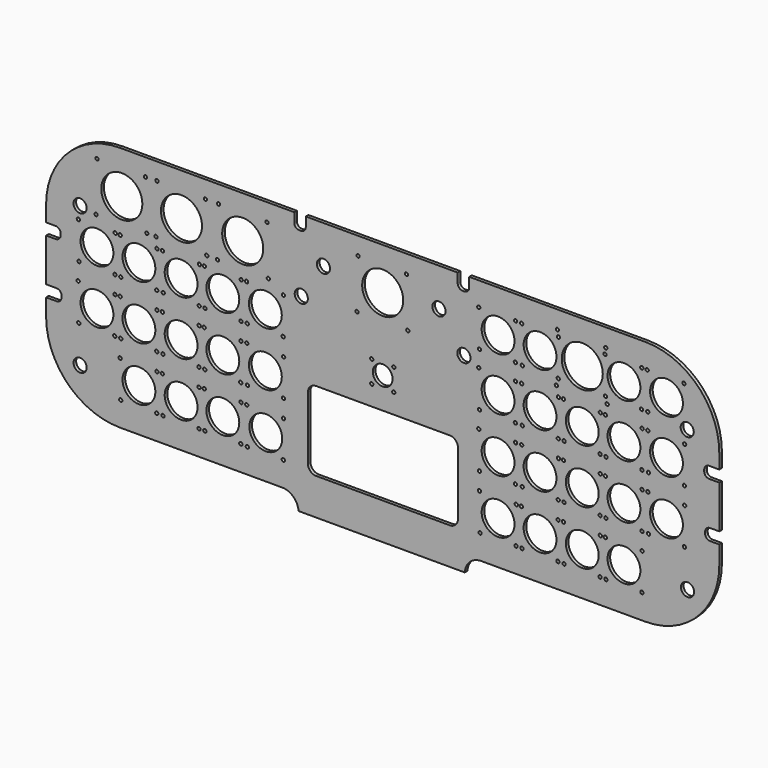
from build123d import *

# Parameters (mm, degrees)
F0_W           = 410
F0_H           = 150
F1_DEPTH       = 1
F1_DEPTH_BACK  = 1
F2_R           = 45
F3_R           = 45
F4_R           = 45
F5_W           = 101.2708619237
F5_H           = 20.8901241422
F6_DEPTH       = 1
F6_DEPTH_BACK  = 1
F7_T1_DEPTH    = 2
F8_T1_DEPTH    = 2
F13_R          = 4
F14_DEPTH      = 28.48665
F14_DEPTH_BACK = 25
F9_R           = 12.5
F9_R_2         = 6
F9_R_3         = 10
F9_W           = 91.4226509631
F9_H           = 48.2046687976
F15_DEPTH      = 25
F15_DEPTH_BACK = 25
F16_DEPTH      = 50
F16_DEPTH_BACK = 50
F19_D          = 2
F19_DEPTH      = 20
F19_TIP        = 0.600860619
F20_D          = 2
F20_DEPTH      = 20
F20_TIP        = 0.600860619
F21_D          = 2
F21_DEPTH      = 20
F21_TIP        = 0.600860619
F22_R          = 5


# Not quite as in the source:
# - a fillet or chamfer that OpenCascade refuses, or shapes differently, is made with other operations: its cross-section is extruded or revolved along the edge and cut away or added


with BuildPart() as f1:
    # F0 (on Front) → F1 (new body, two sides)
    with BuildSketch(Plane.XZ) as f1_sk:
        Rectangle(F0_W, F0_H)
    extrude(amount=F1_DEPTH)
    extrude(f1_sk.sketch, amount=-F1_DEPTH_BACK)

    # F2
    f2_edges = [f1.edges().sort_by_distance(p)[0] for p in [
        (-205, 0, 75),
        (-205, 0, -75),
    ]]
    fillet(f2_edges, radius=F2_R)

    # F3
    f3_edges = [f1.edges().sort_by_distance(p)[0] for p in [
        (205, 0, 75),
    ]]
    fillet(f3_edges, radius=F3_R)

    # F4
    f4_edges = [f1.edges().sort_by_distance(p)[0] for p in [
        (205, 0, -75),
    ]]
    fillet(f4_edges, radius=F4_R)

    # F5 (on Front) → F6 (join, two sides)
    with BuildSketch(Plane.XZ) as f6_sk:
        with Locations((-0.6414987147, -73.9290080965)):
            Rectangle(F5_W, F5_H)
    extrude(amount=F6_DEPTH)
    extrude(f6_sk.sketch, amount=-F6_DEPTH_BACK)

    # F7: fillet of radius 10 on 1 edges, made by hand

    # F7_s2 → F7_t1 (join)
    with BuildSketch(Plane.XZ.offset(-1)):
        with BuildLine():
            ThreePointArc((-61.2573210439, -75), (-54.4111286103, -77.7109912085), (-51.2769296765, -84.3740701675))
            Line((-51.2769296765, -84.3740701675), (-51.2769296765, -75))
            Line((-51.2769296765, -75), (-61.2573210439, -75))
        make_face()
    extrude(amount=F7_T1_DEPTH)

    # F8: fillet of radius 10 on 1 edges, made by hand

    # F8_s2 → F8_t1 (join)
    with BuildSketch(Plane.XZ.offset(-1)):
        with BuildLine():
            ThreePointArc((49.9939322472, -84.3740701675), (53.1281311809, -77.7109912085), (59.9743236145, -75))
            Line((59.9743236145, -75), (49.9939322472, -75))
            Line((49.9939322472, -75), (49.9939322472, -84.3740701675))
        make_face()
    extrude(amount=F8_T1_DEPTH)

    # F13 (on offset) → F14 (cut, two sides)
    with BuildSketch(Plane.XZ.offset(-1)) as f14_sk:
        with Locations((-184.3019276857, 36.01404652)):
            Circle(F13_R)
        with Locations((-184.2796504498, -49.4647398591)):
            Circle(F13_R)
        with Locations((-36.0691249371, 51.8314018846)):
            Circle(F13_R)
        with Locations((-49.5743155479, 31.3860401511)):
            Circle(F13_R)
        with Locations((34.2704169452, 51.8314018846)):
            Circle(F13_R)
        with Locations((49.4637563825, 31.7611843348)):
            Circle(F13_R)
        with Locations((185.4535341263, 36.2629145384)):
            Circle(F13_R)
        with Locations((185.6411099434, -49.4575425982)):
            Circle(F13_R)
    extrude(amount=F14_DEPTH, mode=Mode.SUBTRACT)
    extrude(f14_sk.sketch, amount=-F14_DEPTH_BACK, mode=Mode.SUBTRACT)

    # F9 (on Front) → F15 (cut, two sides)
    with BuildSketch(Plane.XZ) as f15_sk:
        with Locations((0, 49.3269376457)):
            Circle(F9_R)
        with Locations((0, 5.0263302401)):
            Circle(F9_R_2)
        with Locations((-158.883143139, 49.3269376457)):
            Circle(F9_R)
        with Locations((-122.5375886227, 49.3269376457)):
            Circle(F9_R)
        with Locations((-85.2427311078, 49.3269376457)):
            Circle(F9_R)
        with Locations((172.8430779376, 17.2050477801)):
            Circle(F9_R_3)
        with Locations((172.8430779376, -15.7630319912)):
            Circle(F9_R_3)
        with Locations((146.9427224634, -48.7311117624)):
            Circle(F9_R_3)
        with Locations((146.9427224634, 17.2050477801)):
            Circle(F9_R_3)
        with Locations((146.9427224634, -15.7630319912)):
            Circle(F9_R_3)
        with Locations((121.5410116401, -48.7311117624)):
            Circle(F9_R_3)
        with Locations((121.5410116401, 17.2050477801)):
            Circle(F9_R_3)
        with Locations((121.5410116401, -15.7630319912)):
            Circle(F9_R_3)
        with Locations((95.8335487816, -48.7311117624)):
            Circle(F9_R_3)
        with Locations((95.8335487816, 17.2050477801)):
            Circle(F9_R_3)
        with Locations((95.8335487816, -15.7630319912)):
            Circle(F9_R_3)
        with Locations((70.2727413384, -48.7311117624)):
            Circle(F9_R_3)
        with Locations((70.2727413384, 17.2050477801)):
            Circle(F9_R_3)
        with Locations((70.2727413384, -15.7630319912)):
            Circle(F9_R_3)
        with Locations((172.8430779376, 49.4541965136)):
            Circle(F9_R_3)
        with Locations((146.9427224634, 49.4541965136)):
            Circle(F9_R_3)
        with Locations((121.5410116401, 49.4541965136)):
            Circle(F9_R)
        with Locations((95.8335487816, 49.4541965136)):
            Circle(F9_R_3)
        with Locations((70.2727413384, 49.4541965136)):
            Circle(F9_R_3)
        with Locations((-71.4465556458, 17.2050477801)):
            Circle(F9_R_3)
        with Locations((-71.4465556458, -15.7630319912)):
            Circle(F9_R_3)
        with Locations((-97.3469263927, -48.7311117624)):
            Circle(F9_R_3)
        with Locations((-97.3469263927, 17.2050477801)):
            Circle(F9_R_3)
        with Locations((-97.3469263927, -15.7630319912)):
            Circle(F9_R_3)
        with Locations((-122.7486547945, -48.7311117624)):
            Circle(F9_R_3)
        with Locations((-122.7486547945, 17.2050477801)):
            Circle(F9_R_3)
        with Locations((-122.7486547945, -15.7630319912)):
            Circle(F9_R_3)
        with Locations((-148.4561388125, -48.7311117624)):
            Circle(F9_R_3)
        with Locations((-148.4561388125, 17.2050477801)):
            Circle(F9_R_3)
        with Locations((-148.4561388125, -15.7630319912)):
            Circle(F9_R_3)
        with Locations((-174.0169717099, 17.2050477801)):
            Circle(F9_R_3)
        with Locations((-174.0169717099, -15.7630319912)):
            Circle(F9_R_3)
        with Locations((-71.195551245, -48.846316319)):
            Circle(F9_R_3)
        with Locations((0.1603271812, -37.9611137323)):
            Rectangle(F9_W, F9_H)
    extrude(amount=F15_DEPTH, mode=Mode.SUBTRACT)
    extrude(f15_sk.sketch, amount=-F15_DEPTH_BACK, mode=Mode.SUBTRACT)

    # F11 (on offset) → F16 (cut, two sides)
    with BuildSketch(Plane.XZ.offset(1)) as f16_sk:
        with BuildLine():
            Line((-199.1314905395, 20.3550893723), (-210.3814848701, 20.3550893723))
            ThreePointArc((-210.3814848701, 20.3550893723), (-212.5028052137, 19.4764097158), (-213.3814848701, 17.3550893723))
            Line((-213.3814848701, 17.3550893723), (-213.3814848701, 16.3550893723))
            ThreePointArc((-213.3814848701, 16.3550893723), (-212.5028052137, 14.2337690287), (-210.3814848701, 13.3550893723))
            Line((-210.3814848701, 13.3550893723), (-199.1314905395, 13.3550893723))
            ThreePointArc((-199.1314905395, 13.3550893723), (-197.010170196, 14.2337690287), (-196.1314905395, 16.3550893723))
            Line((-196.1314905395, 16.3550893723), (-196.1314905395, 17.3550893723))
            ThreePointArc((-196.1314905395, 17.3550893723), (-197.010170196, 19.4764097158), (-199.1314905395, 20.3550893723))
        make_face()
        with BuildLine():
            Line((-198.5897086968, -12.8095770695), (-209.8397030274, -12.8095770695))
            ThreePointArc((-209.8397030274, -12.8095770695), (-211.961023371, -13.6882567259), (-212.8397030274, -15.8095770695))
            Line((-212.8397030274, -15.8095770695), (-212.8397030274, -16.8095770695))
            ThreePointArc((-212.8397030274, -16.8095770695), (-211.961023371, -18.930897413), (-209.8397030274, -19.8095770695))
            Line((-209.8397030274, -19.8095770695), (-198.5897086968, -19.8095770695))
            ThreePointArc((-198.5897086968, -19.8095770695), (-196.4683883532, -18.930897413), (-195.5897086968, -16.8095770695))
            Line((-195.5897086968, -16.8095770695), (-195.5897086968, -15.8095770695))
            ThreePointArc((-195.5897086968, -15.8095770695), (-196.4683883532, -13.6882567259), (-198.5897086968, -12.8095770695))
        make_face()
        with BuildLine():
            Line((210.0697169493, 21.1949502202), (198.8197226187, 21.1949502202))
            ThreePointArc((198.8197226187, 21.1949502202), (196.6984022751, 20.3162705637), (195.8197226187, 18.1949502202))
            Line((195.8197226187, 18.1949502202), (195.8197226187, 17.1949502202))
            ThreePointArc((195.8197226187, 17.1949502202), (196.6984022751, 15.0736298766), (198.8197226187, 14.1949502202))
            Line((198.8197226187, 14.1949502202), (210.0697169493, 14.1949502202))
            ThreePointArc((210.0697169493, 14.1949502202), (212.1910372928, 15.0736298766), (213.0697169493, 17.1949502202))
            Line((213.0697169493, 17.1949502202), (213.0697169493, 18.1949502202))
            ThreePointArc((213.0697169493, 18.1949502202), (212.1910372928, 20.3162705637), (210.0697169493, 21.1949502202))
        make_face()
        with BuildLine():
            Line((210.611498792, -11.9697162216), (199.3615044614, -11.9697162216))
            ThreePointArc((199.3615044614, -11.9697162216), (197.2401841178, -12.848395878), (196.3615044614, -14.9697162216))
            Line((196.3615044614, -14.9697162216), (196.3615044614, -15.9697162216))
            ThreePointArc((196.3615044614, -15.9697162216), (197.2401841178, -18.0910365651), (199.3615044614, -18.9697162216))
            Line((199.3615044614, -18.9697162216), (210.611498792, -18.9697162216))
            ThreePointArc((210.611498792, -18.9697162216), (212.7328191355, -18.0910365651), (213.611498792, -15.9697162216))
            Line((213.611498792, -15.9697162216), (213.611498792, -14.9697162216))
            ThreePointArc((213.611498792, -14.9697162216), (212.7328191355, -12.848395878), (210.611498792, -11.9697162216))
        make_face()
        with BuildLine():
            Line((-49.8431804255, 85.1224669314), (-50.8431804255, 85.1224669314))
            ThreePointArc((-50.8431804255, 85.1224669314), (-52.964500769, 84.2437872749), (-53.8431804255, 82.1224669314))
            Line((-53.8431804255, 82.1224669314), (-53.8431804255, 69.3415574527))
            ThreePointArc((-53.8431804255, 69.3415574527), (-52.964500769, 67.2202371091), (-50.8431804255, 66.3415574527))
            Line((-50.8431804255, 66.3415574527), (-49.8431804255, 66.3415574527))
            ThreePointArc((-49.8431804255, 66.3415574527), (-47.7218600819, 67.2202371091), (-46.8431804255, 69.3415574527))
            Line((-46.8431804255, 69.3415574527), (-46.8431804255, 82.1224669314))
            ThreePointArc((-46.8431804255, 82.1224669314), (-47.7218600819, 84.2437872749), (-49.8431804255, 85.1224669314))
        make_face()
        with BuildLine():
            Line((49.6914108768, 84.9684671557), (48.6914108768, 84.9684671557))
            ThreePointArc((48.6914108768, 84.9684671557), (46.5700905333, 84.0897874993), (45.6914108768, 81.9684671557))
            Line((45.6914108768, 81.9684671557), (45.6914108768, 69.187557677))
            ThreePointArc((45.6914108768, 69.187557677), (46.5700905333, 67.0662373335), (48.6914108768, 66.187557677))
            Line((48.6914108768, 66.187557677), (49.6914108768, 66.187557677))
            ThreePointArc((49.6914108768, 66.187557677), (51.8127312204, 67.0662373335), (52.6914108768, 69.187557677))
            Line((52.6914108768, 69.187557677), (52.6914108768, 81.9684671557))
            ThreePointArc((52.6914108768, 81.9684671557), (51.8127312204, 84.0897874993), (49.6914108768, 84.9684671557))
        make_face()
    extrude(amount=-F16_DEPTH, mode=Mode.SUBTRACT)
    extrude(f16_sk.sketch, amount=F16_DEPTH_BACK, mode=Mode.SUBTRACT)

    # F19
    with Locations(Plane(origin=(0, 1, 0), x_dir=(-1, 0, 0), z_dir=(0, 1, 0))):
        with Locations((173.9457249641, 64.6309927106), (144.4697678089, 64.4204467535), (137.4428961426, 64.6046726033), (107.9669389874, 64.3941266462), (99.9663267285, 64.3941303715), (70.4903695732, 64.1835844144), (69.648200646, 34.2865427956), (100.5979571491, 34.2865427956), (107.1247700602, 34.4970850274), (138.0745265633, 34.4970850274), (143.6275988817, 34.5234051347), (174.5773553848, 34.5234051347), (185.3234618902, 28.3782370389), (184.9478930235, 5.9693413787), (163.0397588015, 6.0945306905), (162.9145741463, 28.3782370389), (159.8875951022, 28.25988736), (159.5120262355, 5.8509916998), (137.6038920134, 5.9761810116), (137.4787073582, 28.25988736), (134.0318378061, 28.2598854974), (133.6562689394, 5.8509898372), (111.7481347173, 5.976179149), (111.6229500622, 28.2598854974), (108.5976790637, 28.25988736), (108.2221101969, 5.8509916998), (86.3139759749, 5.9761810116), (86.1887913197, 28.25988736), (82.8824583441, 28.4004071727), (82.5068894774, 5.9915115125), (60.5987552553, 6.1167008244), (60.4735706002, 28.4004071727), (185.4622941464, -4.6218661591), (163.0534064025, -4.6218661591), (185.0867252797, -27.0307618193), (163.1785910577, -26.9055725075), (159.5120262355, -27.0307627507), (159.8875951022, -4.6218670905), (137.4787073582, -4.6218670905), (137.6038920134, -26.9055734389), (134.1723632067, -4.6218661591), (111.7634754628, -4.6218661591), (111.888660118, -26.9055725075), (108.362628147, -27.0307613537), (108.7381970137, -4.6218656935), (86.3293092698, -4.6218656935), (86.454493925, -26.9055720419), (82.7419366688, -4.6218666248), (82.366367802, -27.030762285), (60.45823358, -26.9055729732), (60.3330489248, -4.6218666248), (133.79679434, -27.0307618193)):
            Hole(F19_D / 2, depth=F19_DEPTH)
            with Locations((0, 0, -(F19_DEPTH + F19_TIP / 2))):  # 118° drill point
                Cone(0, F19_D / 2, F19_TIP, mode=Mode.SUBTRACT)

    # F20
    with Locations(Plane(origin=(0, 1, 0), x_dir=(-1, 0, 0), z_dir=(0, 1, 0))):
        with Locations((159.9020902067, -37.6898674294), (159.52652134, -60.0987630896), (137.4932024628, -37.6898674294), (137.618387118, -59.9735737778), (134.2047061771, -37.6898655668), (133.8291373104, -60.098761227), (111.9210030884, -59.9735719152), (111.7958184332, -37.6898655668), (108.6949091405, -37.502293475), (108.3193402737, -59.9111891352), (86.4112060517, -59.7859998234), (86.2860213965, -37.502293475), (82.8099455684, -37.6898618415), (82.4343767017, -60.0987575017), (60.4010578245, -37.6898618415), (60.5262424797, -59.9735681899), (15.0090213865, 64.2007170245), (15.6406518072, 34.0931294486), (-15.3091046959, 34.0931294486), (-14.4669357687, 63.9901710674), (-58.954032138, -37.7252576873), (-59.3296010047, -60.1341533475), (-81.3629198819, -37.7252576873), (-81.2377352268, -60.0089640357), (-84.8052520305, -60.1341477595), (-84.4296831638, -37.7252520993), (-106.8385709077, -37.7252520993), (-106.7133862525, -60.0089584477), (-110.4914490134, -60.1341440342), (-110.1158801466, -37.725248374), (-132.5247678906, -37.725248374), (-132.3995832354, -60.0089547224), (-135.9671074897, -60.1341477595), (-135.591538623, -37.7252520993), (-158.0004263669, -37.7252520993), (-157.8752417117, -60.0089584477), (6.6658239812, 11.6348657757), (-6.8047614768, 11.6348657757), (6.6658239812, -1.717556268), (-6.7456797697, -1.7766378587)):
            Hole(F20_D / 2, depth=F20_DEPTH)
            with Locations((0, 0, -(F20_DEPTH + F20_TIP / 2))):  # 118° drill point
                Cone(0, F20_D / 2, F20_TIP, mode=Mode.SUBTRACT)

    # F21
    with Locations(Plane(origin=(0, 1, 0), x_dir=(-1, 0, 0), z_dir=(0, 1, 0))):
        with Locations((-58.5329327732, 60.5981284752), (-80.9418205172, 60.5981284752), (-58.90850164, 38.1892328151), (-80.816635862, 38.3144221269), (-84.6402216703, 60.3875843808), (-107.0491094142, 60.3875843808), (-85.015790537, 37.9786887206), (-106.923924759, 38.1038780324), (-106.4005214721, 64.2007207498), (-135.8764786273, 63.9901747927), (-105.7688910514, 34.0931331739), (-136.7186475545, 34.0931331739), (-135.756554082, 37.9786887206), (-135.3809852153, 60.3875843808), (-157.7898729593, 60.3875843808), (-157.6646883041, 38.1038780324), (-161.4427436143, 37.9786924459), (-161.0671747476, 60.3875881061), (-183.4760624915, 60.3875881061), (-58.5329476744, 28.1745707616), (-80.9418354183, 28.1745707616), (-58.9085165411, 5.7656751014), (-80.8166507632, 5.8908644132), (-84.6402216703, 28.1745716929), (-107.0491094142, 28.1745716929), (-85.015790537, 5.7656760328), (-106.923924759, 5.8908653446), (-110.1158652455, 28.1745716929), (-132.5247529894, 28.1745716929), (-110.4914341122, 5.7656760328), (-132.3995683342, 5.8908653446), (-135.591538623, 27.9640294611), (-158.0004263669, 27.9640294611), (-135.9671074897, 5.555133801), (-157.8752417117, 5.6803231128), (-161.4882666618, 27.9640294611), (-183.8971544057, 27.9640294611), (-161.8638355285, 5.555133801), (-183.7719697505, 5.6803231128), (-58.5329402238, -4.6700684034), (-58.9085090905, -27.0789640635), (-80.9418279678, -4.6700684034), (-80.8166433126, -26.9537747517), (-84.6402216703, -4.670069553), (-85.015790537, -27.0789652131), (-107.0491094142, -4.670069553), (-106.923924759, -26.9537759013), (-110.115872696, -4.6700704843), (-110.4914415628, -27.0789661445), (-132.52476044, -4.6700704843), (-132.3995757848, -26.9537768327), (-135.5915237218, -4.8806136474), (-135.9670925885, -27.2895093076), (-158.0004114658, -4.8806136474), (-157.8752268106, -27.1643199958), (-161.8638504297, -27.2895093076), (-161.4882815629, -4.8806136474), (-183.8971693069, -4.8806136474), (-183.7719846517, -27.1643199958)):
            Hole(F21_D / 2, depth=F21_DEPTH)
            with Locations((0, 0, -(F21_DEPTH + F21_TIP / 2))):  # 118° drill point
                Cone(0, F21_D / 2, F21_TIP, mode=Mode.SUBTRACT)

    # F22
    f22_edges = [f1.edges().sort_by_distance(p)[0] for p in [
        (-45.550998, 0, -13.858779),
        (45.871653, 0, -13.858779),
        (45.871653, 0, -62.063448),
        (-45.550998, 0, -62.063448),
    ]]
    fillet(f22_edges, radius=F22_R)


solid = f1.part
